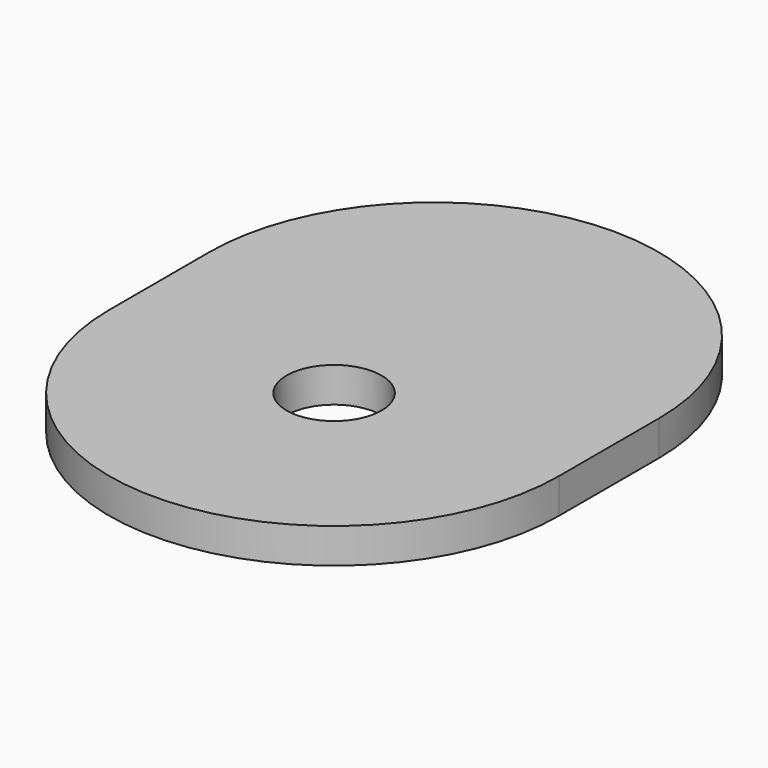
from build123d import *

# Parameters (mm, degrees)
F1_DEPTH  = 7
F2_R      = 9.5
F3_DEPTH  = 10
F6_DEPTH  = 2.5
F4_R      = 5
F7_DEPTH  = 1
F8_W      = 6.5
F8_H      = 4.5
F9_DEPTH  = 2.5
F10_W     = 2
F10_H     = 1.5
F11_DEPTH = 1.5
F12_R     = 44.99999


# Not quite as in the source:
# - a fillet or chamfer is up to 0.001 mm smaller than in the source, because OpenCascade refuses the exact size


with BuildPart() as f1:
    # F0 (on Top) → F1 (new body)
    with BuildSketch(Plane.XY):
        with BuildLine():
            Line((-45, 70), (-45, 0))
            ThreePointArc((-45, 0), (0, -45), (45, 0))
            Line((45, 0), (45, 70))
            Line((45, 70), (-45, 70))
        make_face()
    extrude(amount=F1_DEPTH)

    # F2 (on face) → F3 (cut)
    with BuildSketch(Plane(origin=(0, 0, 0), x_dir=(1, 0, 0), z_dir=(0, 0, -1))):
        Circle(F2_R)
    extrude(amount=-F3_DEPTH, mode=Mode.SUBTRACT)

    # F5 (on face) → F6 (cut)
    with BuildSketch(Plane(origin=(0, 0, 0), x_dir=(1, 0, 0), z_dir=(0, 0, -1))):
        Polygon((20, 32.6008529611), (17.875, 33.8277222831), (15.625, 29.9306079661), (17.75, 28.7037386441), (17.75, 26.25), (22.25, 26.25), (22.25, 28.7037386441), (24.375, 29.9306079661), (22.125, 33.8277222831), align=None)
    extrude(amount=-F6_DEPTH, mode=Mode.SUBTRACT)

    # F4 (on face) → F7 (cut)
    with BuildSketch(Plane(origin=(0, 0, 0), x_dir=(1, 0, 0), z_dir=(0, 0, -1))):
        with Locations((0, -60)):
            Circle(F4_R)
    extrude(amount=-F7_DEPTH, mode=Mode.SUBTRACT)

    # F8 (on face) → F9 (cut)
    with BuildSketch(Plane(origin=(0, 0, 0), x_dir=(1, 0, 0), z_dir=(0, 0, -1))):
        with Locations((-20, 30)):
            Rectangle(F8_W, F8_H)
    extrude(amount=-F9_DEPTH, mode=Mode.SUBTRACT)

    # F10 (on face) → F11 (join)
    with BuildSketch(Plane(origin=(0, 0, 2.5), x_dir=(1, 0, 0), z_dir=(0, 0, -1))):
        with Locations((-20, 31.5)):
            Rectangle(F10_W, F10_H)
        with Locations((-20, 28.5)):
            Rectangle(F10_W, F10_H)
    extrude(amount=F11_DEPTH)

    # F12 (radius 45 in the source; OpenCascade refuses exactly that, so slightly less here)
    f12_edges = [f1.edges().sort_by_distance(p)[0] for p in [
        (-45, 70, 3.5),
        (45, 70, 3.5),
    ]]
    fillet(f12_edges, radius=F12_R)


solid = f1.part
